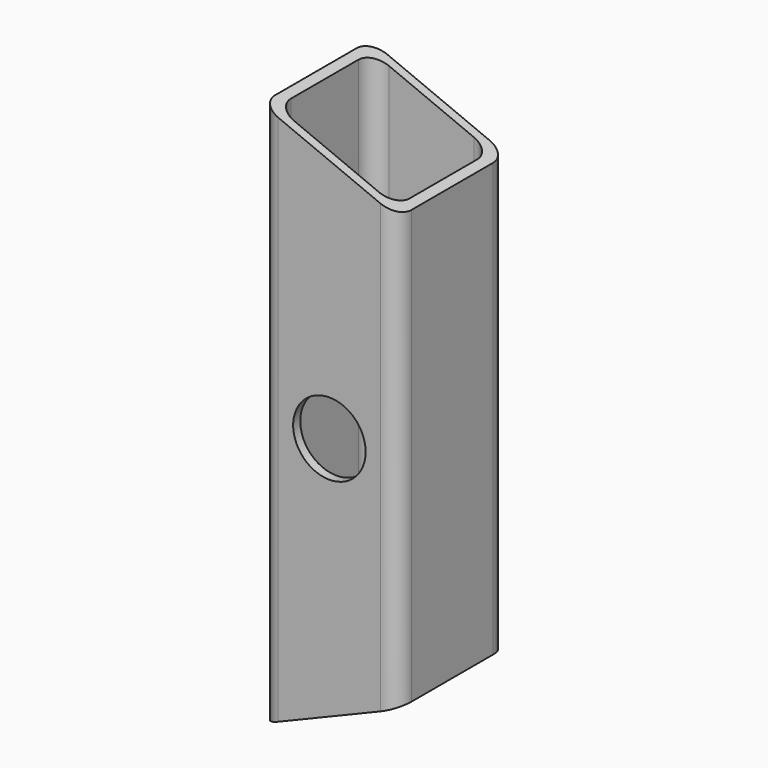
from build123d import *

# Parameters (mm, degrees)
F1_W     = 25.4
F1_H     = 25.4
F2_DEPTH = 101.6
F4_DEPTH = 25.4
F5_R     = 3.175
F6_R     = 6.7437
F7_DEPTH = 25.401


# Not quite as in the source:
# - a variable given as a bare number and used for a length is read in inches; the dataset says mm whatever the document's units were


with BuildPart() as f2:
    # F1 (on Top) → F2 (new body)
    with BuildSketch(Plane.XY):
        Rectangle(F1_W, F1_H)
        with BuildLine():
            ThreePointArc((-11.049, 7.874), (-10.1190640303, 10.1190640303), (-7.874, 11.049))
            Line((-7.874, 11.049), (7.874, 11.049))
            ThreePointArc((7.874, 11.049), (10.1190640303, 10.1190640303), (11.049, 7.874))
            Line((11.049, 7.874), (11.049, -7.874))
            ThreePointArc((11.049, -7.874), (10.1190640303, -10.1190640303), (7.874, -11.049))
            Line((7.874, -11.049), (-7.874, -11.049))
            ThreePointArc((-7.874, -11.049), (-10.1190640303, -10.1190640303), (-11.049, -7.874))
            Line((-11.049, -7.874), (-11.049, 7.874))
        make_face(mode=Mode.SUBTRACT)
    extrude(amount=F2_DEPTH)

    # F3 (on face) → F4 (cut)
    with BuildSketch(Plane.XZ.offset(12.7)):
        Polygon((12.7, 10.5210244843), (-12.7, 0), (12.7, 0), align=None)
        Polygon((12.7, 101.6), (-12.7, 101.6), (12.7, 91.0789755157), align=None)
    extrude(amount=-F4_DEPTH, mode=Mode.SUBTRACT)

    # F5
    f5_edges = [f2.edges().sort_by_distance(p)[0] for p in [
        (-12.7, 12.7, 50.8),
        (12.7, 12.7, 50.8),
        (-12.7, -12.7, 50.8),
        (12.7, -12.7, 50.8),
    ]]
    fillet(f5_edges, radius=F5_R)

    # F6 (on face) → F7 (cut, through all)
    with BuildSketch(Plane.XZ.offset(12.7)):
        with Locations((0, 50.8)):
            Circle(F6_R)
    extrude(amount=-F7_DEPTH, mode=Mode.SUBTRACT)


solid = f2.part
